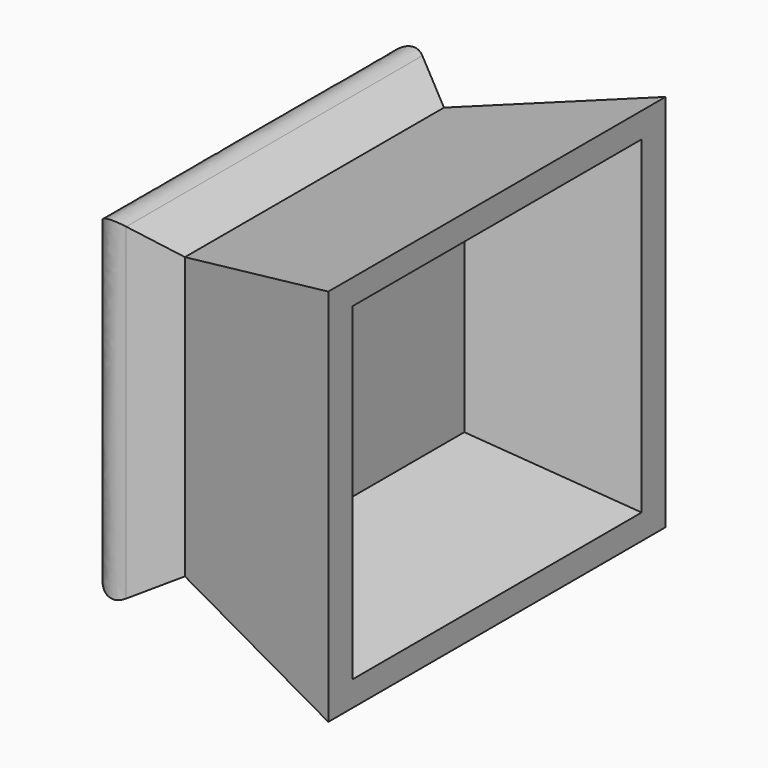
from build123d import *

# Parameters (mm, degrees)
F0_W          = 44.3588159978
F0_H          = 38.4979620576
F1_DEPTH      = 25
F1_TAPER      = -15
F1_DEPTH_BACK = 10
F1_TAPER_BACK = -30
F2_W          = 49.5432667505
F2_H          = 45
F3_DEPTH      = 20
F3_TAPER      = 15
F4_R          = 3
F5_R          = 14.044270733
F6_DEPTH      = 3


with BuildPart() as f1:
    # F0 (on Right) → F1 (new body, two sides)
    with BuildSketch(Plane.YZ) as f1_sk:
        Rectangle(F0_W, F0_H)
    extrude(amount=F1_DEPTH, taper=F1_TAPER)
    extrude(f1_sk.sketch, amount=-F1_DEPTH_BACK, taper=F1_TAPER_BACK)

    # F2 (on face) → F3 (cut)
    with BuildSketch(Plane.YZ.offset(25)):
        Rectangle(F2_W, F2_H)
    extrude(amount=-F3_DEPTH, taper=F3_TAPER, mode=Mode.SUBTRACT)

    # F4
    f4_edges = [f1.edges().sort_by_distance(p)[0] for p in [
        (-10, 27.952911, 0),
        (-10, 0, 25.022484),
        (-10, -27.952911, 0),
        (-10, 0, -25.022484),
    ]]
    fillet(f4_edges, radius=F4_R)

    # F5 (on face) → F6 (cut)
    with BuildSketch(Plane(origin=(-10, 0, 0), x_dir=(0, -1, 0), z_dir=(-1, 0, 0))):
        Circle(F5_R)
    extrude(amount=-F6_DEPTH, mode=Mode.SUBTRACT)


solid = f1.part
